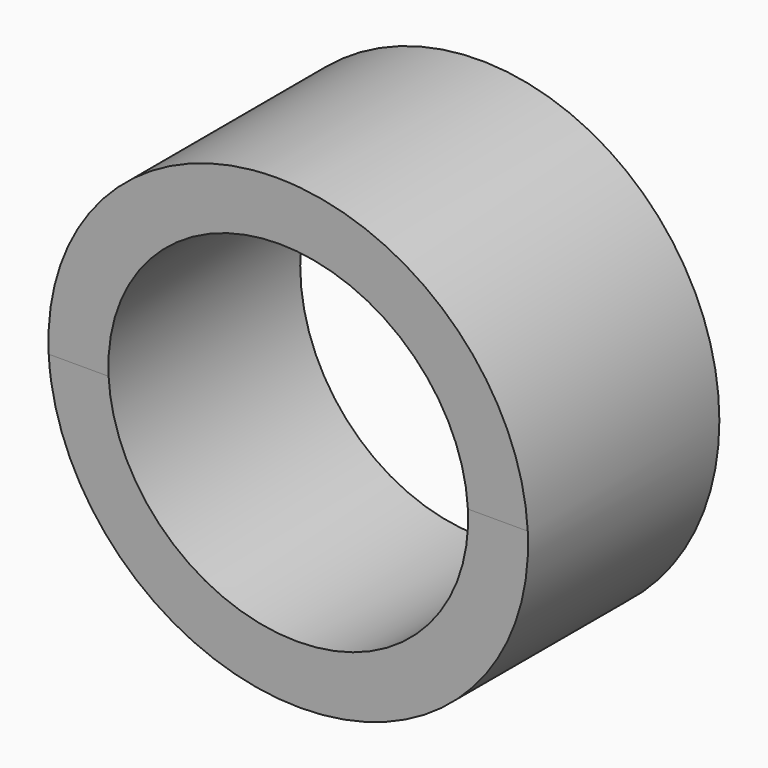
from build123d import *

# Parameters (mm, degrees)
F0_R     = 12.7
F0_R_2   = 9.525
F1_DEPTH = 50.8
F3_DEPTH = 25.4
F4_DEPTH = 25.4


# Not quite as in the source:
# - a feature names something its author has since deleted; it is built from what else it names


with BuildPart() as f1:
    # F0 (on Front) → F1 (new body)
    with BuildSketch(Plane.XZ):
        Circle(F0_R)
        Circle(F0_R_2, mode=Mode.SUBTRACT)
    extrude(amount=F1_DEPTH)

    # F2 (on Right) → F3 (cut)
    with BuildSketch(Plane.YZ):
        Polygon((-36.6640808118, -22.974707012), (-38.1, 0), (-41.275, 50.8), (-42.5002469476, 70.4039511617), (-59.3533739448, 70.4039511617), (-59.3533739448, -22.974707012), align=None)
        Polygon((-38.1, 0), (-12.7, 0), (-15.875, 50.8), (-41.275, 50.8), align=None)
        Polygon((-11.2640808118, -22.974707012), (-12.7, 0), (-38.1, 0), (-36.6640808118, -22.974707012), align=None)
    extrude(amount=-F3_DEPTH, mode=Mode.SUBTRACT)

    # F2 (on Right) → F4 (cut)
    with BuildSketch(Plane.YZ):
        Polygon((-36.6640808118, -22.974707012), (-38.1, 0), (-41.275, 50.8), (-42.5002469476, 70.4039511617), (-59.3533739448, 70.4039511617), (-59.3533739448, -22.974707012), align=None)
        Polygon((-38.1, 0), (-12.7, 0), (-15.875, 50.8), (-41.275, 50.8), align=None)
        Polygon((-11.2640808118, -22.974707012), (-12.7, 0), (-38.1, 0), (-36.6640808118, -22.974707012), align=None)
    extrude(amount=F4_DEPTH, mode=Mode.SUBTRACT)


solid = f1.part
